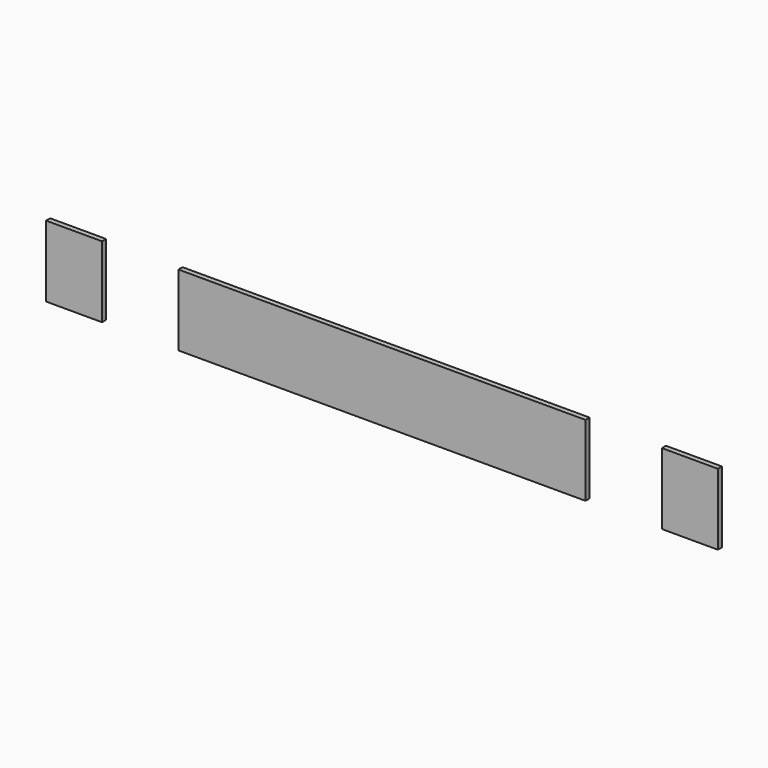
from build123d import *

# Parameters (mm, degrees)
F0_W     = 160.0000202656
F0_H     = 28.0090686734
F0_W_2   = 156
F0_H_2   = 16
F1_DEPTH = 2
F0_W_3   = 22
F2_DEPTH = 2
F3_DEPTH = 2


# Not quite as in the source:
# - a feature names something its author has since deleted; it is built from what else it names


with BuildPart() as f1:
    # F0 (on Front) → F1 (new body)
    with BuildSketch(Plane.XZ):
        with Locations((-4.366838785, 2.9287685109)):
            Rectangle(F0_W, F0_H)
        with Locations((-4.3668536862, -1.0666644891)):
            Rectangle(F0_W_2, F0_H_2, mode=Mode.SUBTRACT)
        with Locations((-4.3668536862, -1.0666644891)):
            Rectangle(F0_W_2, F0_H_2)
    extrude(amount=F1_DEPTH)


with BuildPart() as f2:
    # F0 (on Front) → F2 (new body)
    with BuildSketch(Plane.XZ):
        with Locations((116.6331713478, 2.9287685109)):
            Rectangle(F0_W_3, F0_H)
    extrude(amount=F2_DEPTH)


with BuildPart() as f3:
    # F0 (on Front) → F3 (new body)
    with BuildSketch(Plane.XZ):
        with Locations((-125.3668489178, 2.9287685109)):
            Rectangle(F0_W_3, F0_H)
    extrude(amount=F3_DEPTH)


solid = Compound([f1.part, f2.part, f3.part])
